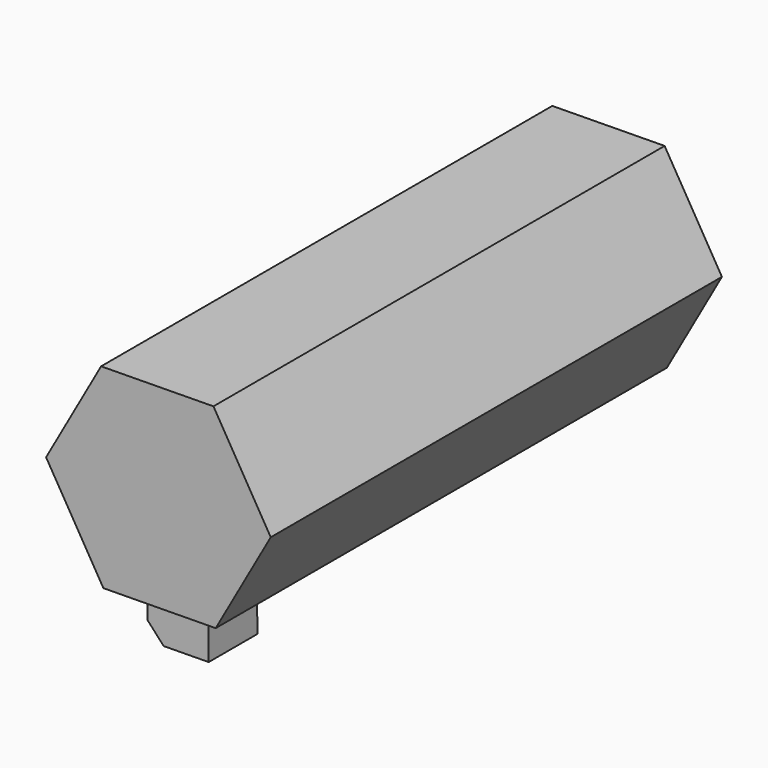
from build123d import *

# Parameters (mm, degrees)
F1_DEPTH = 152.4
F2_W     = 16.4605937898
F2_H     = 16.4605937898
F3_DEPTH = 12.7
F5_DEPTH = 25.4


with BuildPart() as f1:
    # F0 (on Front) → F1 (new body)
    with BuildSketch(Plane.XZ):
        Polygon((15.4824422158, -26.1103501737), (30.3534476601, 0.3530131847), (14.8710054442, 26.4633633584), (-15.4824422158, 26.1103501737), (-30.3534476601, -0.3530131847), (-14.8710054442, -26.4633633584), align=None)
    extrude(amount=F1_DEPTH)

    # F2 (on face) → F3 (join)
    with BuildSketch(Plane(origin=(0.3057183858, 0, -26.2868567661), x_dir=(0.9999323774, 0, 0.0116292988), z_dir=(0.0116292988, 0, -0.9999323774))):
        with Locations((0, 138.0381435156)):
            Rectangle(F2_W, F2_H)
    extrude(amount=F3_DEPTH)

    # F4 (on face) → F5 (cut)
    with BuildSketch(Plane.XZ.offset(146.2684404105)):
        Polygon((-3.4819418117, -39.031766442), (-7.8319489835, -34.2993618355), (-7.7763298602, -39.0817105412), align=None)
    extrude(amount=-F5_DEPTH, mode=Mode.SUBTRACT)


solid = f1.part
